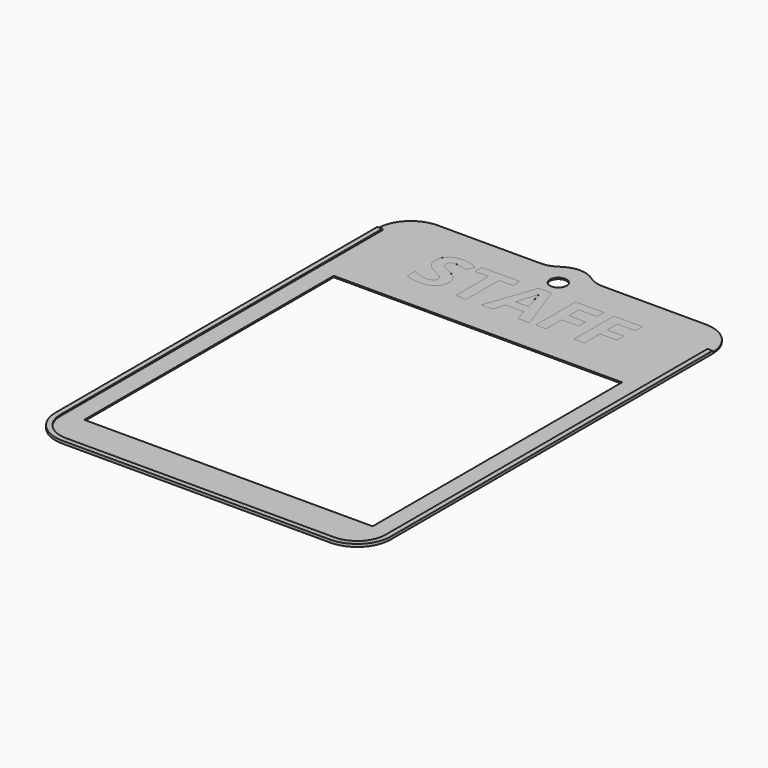
from build123d import *

# Parameters (mm, degrees)
F0_W         = 86
F0_H         = 93
F0_R         = 2.5
F1_DEPTH     = 0.2
F0_TEXT_SIZE = 20.8333333333
F2_DEPTH     = 0.2
F4_DEPTH     = 0.4


# Not quite as in the source:
# - Text() gives the source's letters only with a copy of the font that has no kerning and outlines rounded to 1/6400 em; it was checked with that copy


with BuildPart() as f1:
    # F0 (on Top) → F1 (new body, symmetric)
    with BuildSketch(Plane.XY):
        with BuildLine():
            Line((-9.3273790531, 70), (-40, 70))
            ThreePointArc((-40, 70), (-47.0710678119, 67.0710678119), (-50, 60))
            Line((-50, 60), (-50, -60))
            ThreePointArc((-50, -60), (-47.0710678119, -67.0710678119), (-40, -70))
            Line((-40, -70), (40, -70))
            ThreePointArc((40, -70), (47.0710678119, -67.0710678119), (50, -60))
            Line((50, -60), (50, 60))
            ThreePointArc((50, 60), (47.0710678119, 67.0710678119), (40, 70))
            Line((40, 70), (9.3273790531, 70))
            ThreePointArc((9.3273790531, 70), (6.8778893103, 70.3842268941), (4.6636895265, 71.5))
            ThreePointArc((4.6636895265, 71.5), (0, 73), (-4.6636895265, 71.5))
            ThreePointArc((-4.6636895265, 71.5), (-6.8778893103, 70.3842268941), (-9.3273790531, 70))
        make_face()
        with Locations((0, -11.5)):
            Rectangle(F0_W, F0_H, mode=Mode.SUBTRACT)
        with BuildLine():
            add(Edge.make_bspline(
                [(-20.6705729167, 51.5869140625), (-19.8974609375, 50.5859375), (-19.8974609375, 49.130859375)],
                knots=[0, 0, 0, 1, 1, 1], degree=2))
            add(Edge.make_bspline(
                [(-19.8974609375, 49.130859375), (-19.8974609375, 47.1158854167), (-21.34765625, 45.9554036458)],
                knots=[0, 0, 0, 1, 1, 1], degree=2))
            add(Edge.make_bspline(
                [(-21.34765625, 45.9554036458), (-22.7978515625, 44.794921875), (-25.3792317708, 44.794921875)],
                knots=[0, 0, 0, 1, 1, 1], degree=2))
            add(Edge.make_bspline(
                [(-25.3792317708, 44.794921875), (-27.7620442708, 44.794921875), (-29.5914713542, 45.693359375)],
                knots=[0, 0, 0, 1, 1, 1], degree=2))
            Line((-29.5914713542, 45.693359375), (-29.5914713542, 48.623046875))
            add(Edge.make_bspline(
                [(-29.5914713542, 48.623046875), (-28.0875651042, 47.94921875), (-27.0442708333, 47.67578125)],
                knots=[0, 0, 0, 1, 1, 1], degree=2))
            add(Edge.make_bspline(
                [(-27.0442708333, 47.67578125), (-26.0009765625, 47.40234375), (-25.1350911458, 47.40234375)],
                knots=[0, 0, 0, 1, 1, 1], degree=2))
            add(Edge.make_bspline(
                [(-25.1350911458, 47.40234375), (-24.0999348958, 47.40234375), (-23.544921875, 47.7978515625)],
                knots=[0, 0, 0, 1, 1, 1], degree=2))
            add(Edge.make_bspline(
                [(-23.544921875, 47.7978515625), (-22.9899088542, 48.193359375), (-22.9899088542, 48.9778645833)],
                knots=[0, 0, 0, 1, 1, 1], degree=2))
            add(Edge.make_bspline(
                [(-22.9899088542, 48.9778645833), (-22.9899088542, 49.4140625), (-23.2340494792, 49.755859375)],
                knots=[0, 0, 0, 1, 1, 1], degree=2))
            add(Edge.make_bspline(
                [(-23.2340494792, 49.755859375), (-23.4781901042, 50.09765625), (-23.9518229167, 50.4117838542)],
                knots=[0, 0, 0, 1, 1, 1], degree=2))
            add(Edge.make_bspline(
                [(-23.9518229167, 50.4117838542), (-24.4254557292, 50.7259114583), (-25.8805338542, 51.4192708333)],
                knots=[0, 0, 0, 1, 1, 1], degree=2))
            add(Edge.make_bspline(
                [(-25.8805338542, 51.4192708333), (-27.2412109375, 52.060546875), (-27.9231770833, 52.6497395833)],
                knots=[0, 0, 0, 1, 1, 1], degree=2))
            add(Edge.make_bspline(
                [(-27.9231770833, 52.6497395833), (-28.6051432292, 53.2389322917), (-29.0120442708, 54.0234375)],
                knots=[0, 0, 0, 1, 1, 1], degree=2))
            add(Edge.make_bspline(
                [(-29.0120442708, 54.0234375), (-29.4189453125, 54.8079427083), (-29.4189453125, 55.8528645833)],
                knots=[0, 0, 0, 1, 1, 1], degree=2))
            add(Edge.make_bspline(
                [(-29.4189453125, 55.8528645833), (-29.4189453125, 57.8287760417), (-28.0810546875, 58.9567057292)],
                knots=[0, 0, 0, 1, 1, 1], degree=2))
            add(Edge.make_bspline(
                [(-28.0810546875, 58.9567057292), (-26.7431640625, 60.0846354167), (-24.3831380208, 60.0846354167)],
                knots=[0, 0, 0, 1, 1, 1], degree=2))
            add(Edge.make_bspline(
                [(-24.3831380208, 60.0846354167), (-23.2242838542, 60.0846354167), (-22.1712239583, 59.8111979167)],
                knots=[0, 0, 0, 1, 1, 1], degree=2))
            add(Edge.make_bspline(
                [(-22.1712239583, 59.8111979167), (-21.1181640625, 59.5377604167), (-19.9690755208, 59.0397135417)],
                knots=[0, 0, 0, 1, 1, 1], degree=2))
            Line((-19.9690755208, 59.0397135417), (-20.9847005208, 56.5852864583))
            add(Edge.make_bspline(
                [(-20.9847005208, 56.5852864583), (-22.1761067708, 57.0735677083), (-22.9541015625, 57.2672526042)],
                knots=[0, 0, 0, 1, 1, 1], degree=2))
            add(Edge.make_bspline(
                [(-22.9541015625, 57.2672526042), (-23.7320963542, 57.4609375), (-24.4840494792, 57.4609375)],
                knots=[0, 0, 0, 1, 1, 1], degree=2))
            add(Edge.make_bspline(
                [(-24.4840494792, 57.4609375), (-25.3792317708, 57.4609375), (-25.8577473958, 57.0442708333)],
                knots=[0, 0, 0, 1, 1, 1], degree=2))
            add(Edge.make_bspline(
                [(-25.8577473958, 57.0442708333), (-26.3362630208, 56.6276041667), (-26.3362630208, 55.95703125)],
                knots=[0, 0, 0, 1, 1, 1], degree=2))
            add(Edge.make_bspline(
                [(-26.3362630208, 55.95703125), (-26.3362630208, 55.5403645833), (-26.142578125, 55.2294921875)],
                knots=[0, 0, 0, 1, 1, 1], degree=2))
            add(Edge.make_bspline(
                [(-26.142578125, 55.2294921875), (-25.9488932292, 54.9186197917), (-25.52734375, 54.62890625)],
                knots=[0, 0, 0, 1, 1, 1], degree=2))
            add(Edge.make_bspline(
                [(-25.52734375, 54.62890625), (-25.1057942708, 54.3391927083), (-23.5302734375, 53.5872395833)],
                knots=[0, 0, 0, 1, 1, 1], degree=2))
            add(Edge.make_bspline(
                [(-23.5302734375, 53.5872395833), (-21.4436848958, 52.587890625), (-20.6705729167, 51.5869140625)],
                knots=[0, 0, 0, 1, 1, 1], degree=2))
        make_face(mode=Mode.SUBTRACT)
        Polygon((-11.4632161458, 57.2493489583), (-11.4632161458, 45), (-14.6175130208, 45), (-14.6175130208, 57.2493489583), (-18.6572265625, 57.2493489583), (-18.6572265625, 59.873046875), (-7.4267578125, 59.873046875), (-7.4267578125, 57.2493489583), align=None, mode=Mode.SUBTRACT)
        Polygon((7.3649088542, 45), (3.9664713542, 45), (2.8889973958, 48.5416666667), (-2.5341796875, 48.5416666667), (-3.6116536458, 45), (-7.0100911458, 45), (-1.7594401042, 59.9348958333), (2.0947265625, 59.9348958333), align=None, mode=Mode.SUBTRACT)
        Polygon((12.3388671875, 50.87890625), (12.3388671875, 45), (9.2366536458, 45), (9.2366536458, 59.873046875), (17.7620442708, 59.873046875), (17.7620442708, 57.2884114583), (12.3388671875, 57.2884114583), (12.3388671875, 53.4537760417), (17.3844401042, 53.4537760417), (17.3844401042, 50.87890625), align=None, mode=Mode.SUBTRACT)
        Polygon((23.7744140625, 50.87890625), (23.7744140625, 45), (20.6722005208, 45), (20.6722005208, 59.873046875), (29.1975911458, 59.873046875), (29.1975911458, 57.2884114583), (23.7744140625, 57.2884114583), (23.7744140625, 53.4537760417), (28.8199869792, 53.4537760417), (28.8199869792, 50.87890625), align=None, mode=Mode.SUBTRACT)
        with Locations((0, 65)):
            Circle(F0_R, mode=Mode.SUBTRACT)
    extrude(amount=F1_DEPTH, both=True)

    # F3 (on face) → F4 (join)
    with BuildSketch(Plane.XY.offset(0.2)):
        with BuildLine():
            Line((-48.5, -60), (-48.5, 60))
            Line((-48.5, 60), (-50, 60))
            Line((-50, 60), (-50, -60))
            ThreePointArc((-50, -60), (-47.0710678119, -67.0710678119), (-40, -70))
            Line((-40, -70), (40, -70))
            ThreePointArc((40, -70), (47.0710678119, -67.0710678119), (50, -60))
            Line((50, -60), (50, 60))
            Line((50, 60), (48.5, 60))
            Line((48.5, 60), (48.5, -60))
            ThreePointArc((48.5, -60), (46.0104076401, -66.0104076401), (40, -68.5))
            Line((40, -68.5), (-40, -68.5))
            ThreePointArc((-40, -68.5), (-46.0104076401, -66.0104076401), (-48.5, -60))
        make_face()
    extrude(amount=F4_DEPTH)


with BuildPart() as f1b:
    # F0 (on Top) → F1, piece 2 (new body, symmetric)
    with BuildSketch(Plane.XY):
        with BuildLine():
            Line((-1.7399088542, 51.1848958333), (2.1337890625, 51.1848958333))
            add(Edge.make_bspline(
                [(2.1337890625, 51.1848958333), (0.6396484375, 55.99609375), (0.4508463542, 56.6276041667)],
                knots=[0, 0, 0, 1, 1, 1], degree=2))
            add(Edge.make_bspline(
                [(0.4508463542, 56.6276041667), (0.2620442708, 57.2591145833), (0.1806640625, 57.6236979167)],
                knots=[0, 0, 0, 1, 1, 1], degree=2))
            add(Edge.make_bspline(
                [(0.1806640625, 57.6236979167), (-0.1546223958, 56.3216145833), (-1.7399088542, 51.1848958333)],
                knots=[0, 0, 0, 1, 1, 1], degree=2))
        make_face()
    extrude(amount=F1_DEPTH, both=True)


with BuildPart() as f2:
    # F0 (on Top) → F2 (new body, through all)
    with BuildSketch(Plane.XY):
        with Locations((-30.5485026042, 45)):
            Text('STAFF', F0_TEXT_SIZE, font='Open Sans', font_style=FontStyle.BOLD, text_align=(TextAlign.LEFT, TextAlign.BOTTOM))
    extrude(amount=F2_DEPTH)


solid = Compound([f1.part, f1b.part, f2.part])
